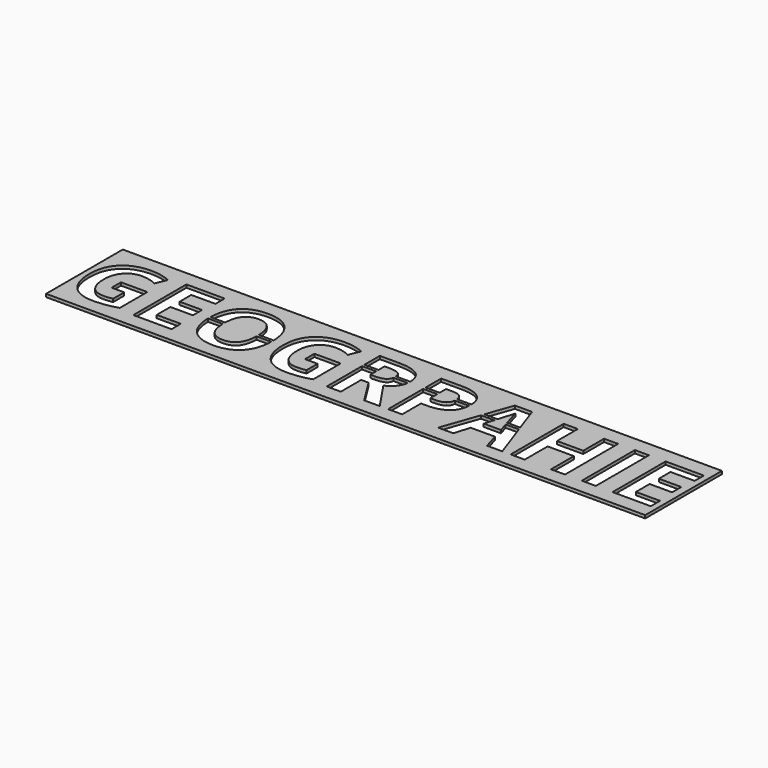
from build123d import *

# Parameters (mm, degrees)
F0_W     = 200
F0_H     = 32
F0_W_2   = 4.6989792207
F0_H_2   = 22.1564871615
F0_H_3   = 1
F1_DEPTH = 1


# Not quite as in the source:
# - a feature names something its author has since deleted; it is built from what else it names


with BuildPart() as f1:
    # F0 (on Top) → F1 (new body)
    with BuildSketch(Plane.XY):
        with Locations((100, 16)):
            Rectangle(F0_W, F0_H)
        with BuildLine():
            Line((11.1970516209, 13.3571272701), (11.1970516209, 17.2705186335))
            Line((11.1970516209, 17.2705186335), (19.9888465921, 17.2705186335))
            Line((19.9888465921, 17.2705186335), (19.9888465921, 5.7825085469))
            add(Edge.make_bspline(
                [(19.9888465921, 5.7825085469), (17.8503018694, 5.0842082293), (15.9639211503, 4.8029483791)],
                knots=[0, 0, 0, 1, 1, 1], degree=2))
            add(Edge.make_bspline(
                [(15.9639211503, 4.8029483791), (14.0775404311, 4.521688529), (12.10872148, 4.521688529)],
                knots=[0, 0, 0, 1, 1, 1], degree=2))
            add(Edge.make_bspline(
                [(12.10872148, 4.521688529), (7.0945372548, 4.521688529), (4.449239871, 7.4700676478)],
                knots=[0, 0, 0, 1, 1, 1], degree=2))
            add(Edge.make_bspline(
                [(4.449239871, 7.4700676478), (1.8039424872, 10.4184467667), (1.8039424872, 15.9369589991)],
                knots=[0, 0, 0, 1, 1, 1], degree=2))
            add(Edge.make_bspline(
                [(1.8039424872, 15.9369589991), (1.8039424872, 21.3002933831), (4.8735543001, 24.2995902335)],
                knots=[0, 0, 0, 1, 1, 1], degree=2))
            add(Edge.make_bspline(
                [(4.8735543001, 24.2995902335), (7.943166113, 27.2988870839), (13.3792401135, 27.2988870839)],
                knots=[0, 0, 0, 1, 1, 1], degree=2))
            add(Edge.make_bspline(
                [(13.3792401135, 27.2988870839), (16.7931527774, 27.2988870839), (19.9597507456, 25.9362316029)],
                knots=[0, 0, 0, 1, 1, 1], degree=2))
            Line((19.9597507456, 25.9362316029), (18.3982736464, 22.1780180879))
            add(Edge.make_bspline(
                [(18.3982736464, 22.1780180879), (15.9736197658, 23.3903450282), (13.3501442669, 23.3903450282)],
                knots=[0, 0, 0, 1, 1, 1], degree=2))
            add(Edge.make_bspline(
                [(13.3501442669, 23.3903450282), (10.3047789928, 23.3903450282), (8.471740659, 21.343937153)],
                knots=[0, 0, 0, 1, 1, 1], degree=2))
            add(Edge.make_bspline(
                [(8.471740659, 21.343937153), (6.6387023252, 19.2975292777), (6.6387023252, 15.8448221516)],
                knots=[0, 0, 0, 1, 1, 1], degree=2))
            add(Edge.make_bspline(
                [(6.6387023252, 15.8448221516), (6.6387023252, 12.2369371772), (8.1153165386, 10.3360085348)],
                knots=[0, 0, 0, 1, 1, 1], degree=2))
            add(Edge.make_bspline(
                [(8.1153165386, 10.3360085348), (9.5919307519, 8.4350798923), (12.4093785612, 8.4350798923)],
                knots=[0, 0, 0, 1, 1, 1], degree=2))
            add(Edge.make_bspline(
                [(12.4093785612, 8.4350798923), (13.8835681207, 8.4350798923), (15.3965521422, 8.7357369735)],
                knots=[0, 0, 0, 1, 1, 1], degree=2))
            Line((15.3965521422, 8.7357369735), (15.3965521422, 13.3571272701))
            Line((15.3965521422, 13.3571272701), (11.1970516209, 13.3571272701))
        make_face(mode=Mode.SUBTRACT)
        Polygon((38.0185728487, 8.706641127), (38.0185728487, 4.8271949179), (25.2600441287, 4.8271949179), (25.2600441287, 26.9836820794), (38.0185728487, 26.9836820794), (38.0185728487, 23.1333317169), (29.9590233494, 23.1333317169), (29.9590233494, 18.2694760323), (37.4609024562, 18.2694760323), (37.4609024562, 14.4191256698), (29.9590233494, 14.4191256698), (29.9590233494, 8.706641127), align=None, mode=Mode.SUBTRACT)
        with BuildLine():
            add(Edge.make_bspline(
                [(41.6555536697, 15.9660548457), (41.6555536697, 16.236144344), (41.6620706058, 16.5)],
                knots=[0, 0, 0, 0.048813765, 0.048813765, 0.048813765], degree=2))
            add(Edge.make_bspline(
                [(41.6620706058, 16.5), (41.7890597846, 21.6414978525), (44.3905632471, 24.4159736198)],
                knots=[0.048813765, 0.048813765, 0.048813765, 1, 1, 1], degree=2))
            add(Edge.make_bspline(
                [(44.3905632471, 24.4159736198), (47.1255728245, 27.3328322382), (52.2318938971, 27.3328322382)],
                knots=[0, 0, 0, 1, 1, 1], degree=2))
            add(Edge.make_bspline(
                [(52.2318938971, 27.3328322382), (57.3382149698, 27.3328322382), (60.0441287006, 24.391727081)],
                knots=[0, 0, 0, 1, 1, 1], degree=2))
            add(Edge.make_bspline(
                [(60.0441287006, 24.391727081), (62.61019587, 21.6026236075), (62.7428149058, 16.5)],
                knots=[0, 0, 0, 0.9483181744, 0.9483181744, 0.9483181744], degree=2))
            add(Edge.make_bspline(
                [(62.7428149058, 16.5), (62.7500424314, 16.2219151647), (62.7500424314, 15.9369589991)],
                knots=[0.9483181744, 0.9483181744, 0.9483181744, 1, 1, 1], degree=2))
            add(Edge.make_bspline(
                [(62.7500424314, 15.9369589991), (62.7500424314, 15.7164340599), (62.7456635168, 15.5)],
                knots=[0, 0, 0, 0.0400665642, 0.0400665642, 0.0400665642], degree=2))
            add(Edge.make_bspline(
                [(62.7456635168, 15.5), (62.6407514373, 10.3145718262), (60.0223068157, 7.4773416095)],
                knots=[0.0400665642, 0.0400665642, 0.0400665642, 1, 1, 1], degree=2))
            add(Edge.make_bspline(
                [(60.0223068157, 7.4773416095), (57.2945712, 4.521688529), (52.2027980506, 4.521688529)],
                knots=[0, 0, 0, 1, 1, 1], degree=2))
            add(Edge.make_bspline(
                [(52.2027980506, 4.521688529), (47.1110249012, 4.521688529), (44.3832892855, 7.4773416095)],
                knots=[0, 0, 0, 1, 1, 1], degree=2))
            add(Edge.make_bspline(
                [(44.3832892855, 7.4773416095), (41.7715830671, 10.3072703918), (41.6604891998, 15.5)],
                knots=[0, 0, 0, 0.9574631072, 0.9574631072, 0.9574631072], degree=2))
            add(Edge.make_bspline(
                [(41.6604891998, 15.5), (41.6555536697, 15.7306956591), (41.6555536697, 15.9660548457)],
                knots=[0.9574631072, 0.9574631072, 0.9574631072, 1, 1, 1], degree=2))
        make_face(mode=Mode.SUBTRACT)
        with BuildLine():
            Line((75.7510365395, 13.3571272701), (75.7510365395, 17.2705186335))
            Line((75.7510365395, 17.2705186335), (84.5428315108, 17.2705186335))
            Line((84.5428315108, 17.2705186335), (84.5428315108, 5.7825085469))
            add(Edge.make_bspline(
                [(84.5428315108, 5.7825085469), (82.4042867881, 5.0842082293), (80.5179060689, 4.8029483791)],
                knots=[0, 0, 0, 1, 1, 1], degree=2))
            add(Edge.make_bspline(
                [(80.5179060689, 4.8029483791), (78.6315253498, 4.521688529), (76.6627063987, 4.521688529)],
                knots=[0, 0, 0, 1, 1, 1], degree=2))
            add(Edge.make_bspline(
                [(76.6627063987, 4.521688529), (71.6485221735, 4.521688529), (69.0032247897, 7.4700676478)],
                knots=[0, 0, 0, 1, 1, 1], degree=2))
            add(Edge.make_bspline(
                [(69.0032247897, 7.4700676478), (66.3579274059, 10.4184467667), (66.3579274059, 15.9369589991)],
                knots=[0, 0, 0, 1, 1, 1], degree=2))
            add(Edge.make_bspline(
                [(66.3579274059, 15.9369589991), (66.3579274059, 21.3002933831), (69.4275392188, 24.2995902335)],
                knots=[0, 0, 0, 1, 1, 1], degree=2))
            add(Edge.make_bspline(
                [(69.4275392188, 24.2995902335), (72.4971510317, 27.2988870839), (77.9332250321, 27.2988870839)],
                knots=[0, 0, 0, 1, 1, 1], degree=2))
            add(Edge.make_bspline(
                [(77.9332250321, 27.2988870839), (81.3471376961, 27.2988870839), (84.5137356642, 25.9362316029)],
                knots=[0, 0, 0, 1, 1, 1], degree=2))
            Line((84.5137356642, 25.9362316029), (82.9522585651, 22.1780180879))
            add(Edge.make_bspline(
                [(82.9522585651, 22.1780180879), (80.5276046844, 23.3903450282), (77.9041291856, 23.3903450282)],
                knots=[0, 0, 0, 1, 1, 1], degree=2))
            add(Edge.make_bspline(
                [(77.9041291856, 23.3903450282), (74.8587639115, 23.3903450282), (73.0257255777, 21.343937153)],
                knots=[0, 0, 0, 1, 1, 1], degree=2))
            add(Edge.make_bspline(
                [(73.0257255777, 21.343937153), (71.1926872439, 19.2975292777), (71.1926872439, 15.8448221516)],
                knots=[0, 0, 0, 1, 1, 1], degree=2))
            add(Edge.make_bspline(
                [(71.1926872439, 15.8448221516), (71.1926872439, 12.2369371772), (72.6693014572, 10.3360085348)],
                knots=[0, 0, 0, 1, 1, 1], degree=2))
            add(Edge.make_bspline(
                [(72.6693014572, 10.3360085348), (74.1459156705, 8.4350798923), (76.9633634799, 8.4350798923)],
                knots=[0, 0, 0, 1, 1, 1], degree=2))
            add(Edge.make_bspline(
                [(76.9633634799, 8.4350798923), (78.4375530393, 8.4350798923), (79.9505370608, 8.7357369735)],
                knots=[0, 0, 0, 1, 1, 1], degree=2))
            Line((79.9505370608, 8.7357369735), (79.9505370608, 13.3571272701))
            Line((79.9505370608, 13.3571272701), (75.7510365395, 13.3571272701))
        make_face(mode=Mode.SUBTRACT)
        with BuildLine():
            Line((89.8140290474, 19.5501047075), (89.8140290474, 20.5501047075))
            Line((89.8140290474, 20.5501047075), (89.8140290474, 26.9836820794))
            Line((89.8140290474, 26.9836820794), (96.2684576777, 26.9836820794))
            add(Edge.make_bspline(
                [(96.2684576777, 26.9836820794), (100.7880125112, 26.9836820794), (102.9532284266, 25.3397667483)],
                knots=[0, 0, 0, 1, 1, 1], degree=2))
            add(Edge.make_bspline(
                [(102.9532284266, 25.3397667483), (105.0516471946, 23.7465663847), (105.1163836428, 20.5501047075)],
                knots=[0, 0, 0, 0.9691498908, 0.9691498908, 0.9691498908], degree=2))
            add(Edge.make_bspline(
                [(105.1163836428, 20.5501047075), (105.1184443421, 20.4483545109), (105.1184443421, 20.3449797541)],
                knots=[0.9691498908, 0.9691498908, 0.9691498908, 1, 1, 1], degree=2))
            add(Edge.make_bspline(
                [(105.1184443421, 20.3449797541), (105.1184443421, 19.9381923705), (105.0719051499, 19.5501047075)],
                knots=[0, 0, 0, 0.2081530033, 0.2081530033, 0.2081530033], degree=2))
            add(Edge.make_bspline(
                [(105.0719051499, 19.5501047075), (104.8948626908, 18.0737577624), (104.0443226729, 16.8680260893)],
                knots=[0.2081530033, 0.2081530033, 0.2081530033, 1, 1, 1], degree=2))
            add(Edge.make_bspline(
                [(104.0443226729, 16.8680260893), (102.9702010038, 15.3453434522), (100.996532745, 14.4821666707)],
                knots=[0, 0, 0, 1, 1, 1], degree=2))
            add(Edge.make_bspline(
                [(100.996532745, 14.4821666707), (106.0010183546, 7.0093834105), (107.5140023762, 4.8271949179)],
                knots=[0, 0, 0, 1, 1, 1], degree=2))
            Line((107.5140023762, 4.8271949179), (102.3009965327, 4.8271949179))
            Line((102.3009965327, 4.8271949179), (97.0104017651, 13.3280314235))
            Line((97.0104017651, 13.3280314235), (94.5130082681, 13.3280314235))
            Line((94.5130082681, 13.3280314235), (94.5130082681, 4.8271949179))
            Line((94.5130082681, 4.8271949179), (89.8140290474, 4.8271949179))
            Line((89.8140290474, 4.8271949179), (89.8140290474, 19.5501047075))
        make_face(mode=Mode.SUBTRACT)
        with BuildLine():
            Line((110.3023543389, 19.4673790485), (110.3023543389, 20.4673790485))
            Line((110.3023543389, 20.4673790485), (110.3023543389, 26.9836820794))
            Line((110.3023543389, 26.9836820794), (117.3774943627, 26.9836820794))
            add(Edge.make_bspline(
                [(117.3774943627, 26.9836820794), (121.4121184201, 26.9836820794), (123.5094440269, 25.2476299008)],
                knots=[0, 0, 0, 1, 1, 1], degree=2))
            add(Edge.make_bspline(
                [(123.5094440269, 25.2476299008), (125.484854695, 23.6124922842), (125.5996828693, 20.4673790485)],
                knots=[0, 0, 0, 0.9418712391, 0.9418712391, 0.9418712391], degree=2))
            add(Edge.make_bspline(
                [(125.5996828693, 20.4673790485), (125.6067696336, 20.2732744537), (125.6067696336, 20.0734185195)],
                knots=[0.9418712391, 0.9418712391, 0.9418712391, 1, 1, 1], degree=2))
            add(Edge.make_bspline(
                [(125.6067696336, 20.0734185195), (125.6067696336, 19.7641047233), (125.5900699964, 19.4673790485)],
                knots=[0, 0, 0, 0.0864297351, 0.0864297351, 0.0864297351], degree=2))
            add(Edge.make_bspline(
                [(125.5900699964, 19.4673790485), (125.4135532921, 16.3309613193), (123.3712387557, 14.6009747109)],
                knots=[0.0864297351, 0.0864297351, 0.0864297351, 1, 1, 1], degree=2))
            add(Edge.make_bspline(
                [(123.3712387557, 14.6009747109), (121.1357078777, 12.7073200301), (117.0137962806, 12.7073200301)],
                knots=[0, 0, 0, 1, 1, 1], degree=2))
            Line((117.0137962806, 12.7073200301), (115.0013335596, 12.7073200301))
            Line((115.0013335596, 12.7073200301), (115.0013335596, 4.8271949179))
            Line((115.0013335596, 4.8271949179), (110.3023543389, 4.8271949179))
            Line((110.3023543389, 4.8271949179), (110.3023543389, 19.4673790485))
        make_face(mode=Mode.SUBTRACT)
        Polygon((131.3632866146, 17.2284944803), (131.7148559258, 18.2284944803), (134.8253036879, 27.0758189268), (140.5668840773, 27.0758189268), (143.6889020108, 18.2284944803), (144.0417790814, 17.2284944803), (148.4179133429, 4.8271949179), (143.3552360401, 4.8271949179), (141.7501151711, 10.1032417622), (133.6711684407, 10.1032417622), (132.0660475717, 4.8271949179), (127.0033702689, 4.8271949179), align=None, mode=Mode.SUBTRACT)
        Polygon((169.362073564, 26.9836820794), (169.362073564, 4.8271949179), (164.6776422666, 4.8271949179), (164.6776422666, 14.3900298232), (155.9052445263, 14.3900298232), (155.9052445263, 4.8271949179), (151.2062653056, 4.8271949179), (151.2062653056, 26.9836820794), (155.9052445263, 26.9836820794), (155.9052445263, 18.2985718789), (164.6776422666, 18.2985718789), (164.6776422666, 26.9836820794), align=None, mode=Mode.SUBTRACT)
        with Locations((177.3028150232, 15.9054384987)):
            Rectangle(F0_W_2, F0_H_2, mode=Mode.SUBTRACT)
        Polygon((197.9875372791, 8.706641127), (197.9875372791, 4.8271949179), (185.229008559, 4.8271949179), (185.229008559, 26.9836820794), (197.9875372791, 26.9836820794), (197.9875372791, 23.1333317169), (189.9279877797, 23.1333317169), (189.9279877797, 18.2694760323), (197.4298668865, 18.2694760323), (197.4298668865, 14.4191256698), (189.9279877797, 14.4191256698), (189.9279877797, 8.706641127), align=None, mode=Mode.SUBTRACT)
        with BuildLine():
            Line((57.8181957487, 15.5), (46.5874707337, 15.5))
            add(Edge.make_bspline(
                [(46.5874707337, 15.5), (46.6665474848, 12.1102114993), (47.9911742599, 10.3432824964)],
                knots=[0.0596973824, 0.0596973824, 0.0596973824, 1, 1, 1], degree=2))
            add(Edge.make_bspline(
                [(47.9911742599, 10.3432824964), (49.3998981645, 8.4641757389), (52.2027980506, 8.4641757389)],
                knots=[0, 0, 0, 1, 1, 1], degree=2))
            add(Edge.make_bspline(
                [(52.2027980506, 8.4641757389), (57.656350345, 8.4641757389), (57.8181957487, 15.5)],
                knots=[0, 0, 0, 0.9703229391, 0.9703229391, 0.9703229391], degree=2))
        make_face()
        with BuildLine():
            add(Edge.make_bspline(
                [(48.0057221832, 21.5330601557), (46.6925516643, 19.7926058735), (46.5909675604, 16.5)],
                knots=[0, 0, 0, 0.9226421075, 0.9226421075, 0.9226421075], degree=2))
            Line((46.5909675604, 16.5), (57.8149184145, 16.5))
            add(Edge.make_bspline(
                [(57.8149184145, 16.5), (57.6086671178, 23.4194408748), (52.2318938971, 23.4194408748)],
                knots=[0.0383596794, 0.0383596794, 0.0383596794, 1, 1, 1], degree=2))
            add(Edge.make_bspline(
                [(52.2318938971, 23.4194408748), (49.4289940111, 23.4194408748), (48.0057221832, 21.5330601557)],
                knots=[0, 0, 0, 1, 1, 1], degree=2))
        make_face()
        with BuildLine():
            Line((139.6358245633, 17.2284944803), (135.8330191332, 17.2284944803))
            add(Edge.make_bspline(
                [(135.8330191332, 17.2284944803), (135.3919484767, 15.7826706927), (134.8543995345, 14.0408796644)],
                knots=[0.772380585, 0.772380585, 0.772380585, 1, 1, 1], degree=2))
            Line((134.8543995345, 14.0408796644), (140.6250757704, 14.0408796644))
            add(Edge.make_bspline(
                [(140.6250757704, 14.0408796644), (140.0699793007, 15.8283144841), (139.6358245633, 17.2284944803)],
                knots=[0, 0, 0, 0.2493882756, 0.2493882756, 0.2493882756], degree=2))
        make_face()
        with BuildLine():
            Line((120.8436359326, 19.4673790485), (115.0013335596, 19.4673790485))
            Line((115.0013335596, 19.4673790485), (115.0013335596, 16.5576703926))
            Line((115.0013335596, 16.5576703926), (116.5482627355, 16.5576703926))
            add(Edge.make_bspline(
                [(116.5482627355, 16.5576703926), (118.711053997, 16.5576703926), (119.7876003201, 17.4135732124)],
                knots=[0, 0, 0, 1, 1, 1], degree=2))
            add(Edge.make_bspline(
                [(119.7876003201, 17.4135732124), (120.7155507821, 18.1513356293), (120.8436359326, 19.4673790485)],
                knots=[0, 0, 0, 0.8619698402, 0.8619698402, 0.8619698402], degree=2))
        make_face()
        with BuildLine():
            Line((115.0013335596, 23.1333317169), (115.0013335596, 20.4673790485))
            Line((115.0013335596, 20.4673790485), (120.8353082496, 20.4673790485))
            add(Edge.make_bspline(
                [(120.8353082496, 20.4673790485), (120.702866137, 21.6982103624), (119.9621753995, 22.3453192057)],
                knots=[0.1788089224, 0.1788089224, 0.1788089224, 1, 1, 1], degree=2))
            add(Edge.make_bspline(
                [(119.9621753995, 22.3453192057), (119.0602041559, 23.1333317169), (117.1350289746, 23.1333317169)],
                knots=[0, 0, 0, 1, 1, 1], degree=2))
            Line((117.1350289746, 23.1333317169), (115.0013335596, 23.1333317169))
        make_face()
        with BuildLine():
            Line((94.5130082681, 23.1333317169), (94.5130082681, 20.5501047075))
            Line((94.5130082681, 20.5501047075), (100.3634520099, 20.5501047075))
            add(Edge.make_bspline(
                [(100.3634520099, 20.5501047075), (100.2600364504, 21.8710044043), (99.2920010668, 22.4665518997)],
                knots=[0.1068303507, 0.1068303507, 0.1068303507, 1, 1, 1], degree=2))
            add(Edge.make_bspline(
                [(99.2920010668, 22.4665518997), (98.2081807822, 23.1333317169), (95.9387047499, 23.1333317169)],
                knots=[0, 0, 0, 1, 1, 1], degree=2))
            Line((95.9387047499, 23.1333317169), (94.5130082681, 23.1333317169))
        make_face()
        with BuildLine():
            Line((100.3220361566, 19.5501047075), (94.5130082681, 19.5501047075))
            Line((94.5130082681, 19.5501047075), (94.5130082681, 17.1492859394))
            Line((94.5130082681, 17.1492859394), (96.0259922896, 17.1492859394))
            add(Edge.make_bspline(
                [(96.0259922896, 17.1492859394), (98.2566738598, 17.1492859394), (99.3162476057, 17.8912300269)],
                knots=[0, 0, 0, 1, 1, 1], degree=2))
            add(Edge.make_bspline(
                [(99.3162476057, 17.8912300269), (100.137096865, 18.4660123458), (100.3220361566, 19.5501047075)],
                knots=[0, 0, 0, 0.7746976202, 0.7746976202, 0.7746976202], degree=2))
        make_face()
        with BuildLine():
            Line((57.8149184145, 16.5), (46.5909675604, 16.5))
            add(Edge.make_bspline(
                [(46.5909675604, 16.5), (46.5824503552, 16.223935154), (46.5824503552, 15.9369589991)],
                knots=[0.9226421075, 0.9226421075, 0.9226421075, 1, 1, 1], degree=2))
            add(Edge.make_bspline(
                [(46.5824503552, 15.9369589991), (46.5824503552, 15.7152089087), (46.5874707337, 15.5)],
                knots=[0, 0, 0, 0.0596973824, 0.0596973824, 0.0596973824], degree=2))
            Line((46.5874707337, 15.5), (57.8181957487, 15.5))
            add(Edge.make_bspline(
                [(57.8181957487, 15.5), (57.8231457459, 15.715188755), (57.8231457459, 15.9369589991)],
                knots=[0.9703229391, 0.9703229391, 0.9703229391, 1, 1, 1], degree=2))
            add(Edge.make_bspline(
                [(57.8231457459, 15.9369589991), (57.8231457459, 16.2239846046), (57.8149184145, 16.5)],
                knots=[0, 0, 0, 0.0383596794, 0.0383596794, 0.0383596794], degree=2))
        make_face()
        with BuildLine():
            add(Edge.make_bspline(
                [(137.7154911136, 23.6328104163), (137.3705203782, 22.2931182399), (136.1372867158, 18.2284944803)],
                knots=[0, 0, 0, 0.6906615554, 0.6906615554, 0.6906615554], degree=2))
            Line((136.1372867158, 18.2284944803), (139.3258767157, 18.2284944803))
            add(Edge.make_bspline(
                [(139.3258767157, 18.2284944803), (138.3026761722, 21.5311576243), (138.1179836578, 22.1489222414)],
                knots=[0.3433385026, 0.3433385026, 0.3433385026, 1, 1, 1], degree=2))
            add(Edge.make_bspline(
                [(138.1179836578, 22.1489222414), (137.8367238077, 23.089687947), (137.7154911136, 23.6328104163)],
                knots=[0, 0, 0, 1, 1, 1], degree=2))
        make_face()
        with BuildLine():
            Line((120.8353082496, 20.4673790485), (115.0013335596, 20.4673790485))
            Line((115.0013335596, 20.4673790485), (115.0013335596, 19.4673790485))
            Line((115.0013335596, 19.4673790485), (120.8436359326, 19.4673790485))
            add(Edge.make_bspline(
                [(120.8436359326, 19.4673790485), (120.8641466431, 19.6781215535), (120.8641466431, 19.9036927479)],
                knots=[0.8619698402, 0.8619698402, 0.8619698402, 1, 1, 1], degree=2))
            add(Edge.make_bspline(
                [(120.8641466431, 19.9036927479), (120.8641466431, 20.1993736757), (120.8353082496, 20.4673790485)],
                knots=[0, 0, 0, 0.1788089224, 0.1788089224, 0.1788089224], degree=2))
        make_face()
        with BuildLine():
            Line((100.3634520099, 20.5501047075), (94.5130082681, 20.5501047075))
            Line((94.5130082681, 20.5501047075), (94.5130082681, 19.5501047075))
            Line((94.5130082681, 19.5501047075), (100.3220361566, 19.5501047075))
            add(Edge.make_bspline(
                [(100.3220361566, 19.5501047075), (100.3758213515, 19.8653871902), (100.3758213515, 20.2237470601)],
                knots=[0.7746976202, 0.7746976202, 0.7746976202, 1, 1, 1], degree=2))
            add(Edge.make_bspline(
                [(100.3758213515, 20.2237470601), (100.3758213515, 20.392114366), (100.3634520099, 20.5501047075)],
                knots=[0, 0, 0, 0.1068303507, 0.1068303507, 0.1068303507], degree=2))
        make_face()
        with BuildLine():
            Line((46.5909675604, 16.5), (41.6620706058, 16.5))
            add(Edge.make_bspline(
                [(41.6555536697, 15.9660548457), (41.6555536697, 16.236144344), (41.6620706058, 16.5)],
                knots=[0, 0, 0, 0.048813765, 0.048813765, 0.048813765], degree=2))
            add(Edge.make_bspline(
                [(41.6604891998, 15.5), (41.6555536697, 15.7306956591), (41.6555536697, 15.9660548457)],
                knots=[0.9574631072, 0.9574631072, 0.9574631072, 1, 1, 1], degree=2))
            Line((41.6604891998, 15.5), (46.5874707337, 15.5))
            add(Edge.make_bspline(
                [(46.5824503552, 15.9369589991), (46.5824503552, 15.7152089087), (46.5874707337, 15.5)],
                knots=[0, 0, 0, 0.0596973824, 0.0596973824, 0.0596973824], degree=2))
            add(Edge.make_bspline(
                [(46.5909675604, 16.5), (46.5824503552, 16.223935154), (46.5824503552, 15.9369589991)],
                knots=[0.9226421075, 0.9226421075, 0.9226421075, 1, 1, 1], degree=2))
        make_face()
        with BuildLine():
            Line((62.7428149058, 16.5), (57.8149184145, 16.5))
            add(Edge.make_bspline(
                [(57.8231457459, 15.9369589991), (57.8231457459, 16.2239846046), (57.8149184145, 16.5)],
                knots=[0, 0, 0, 0.0383596794, 0.0383596794, 0.0383596794], degree=2))
            add(Edge.make_bspline(
                [(57.8181957487, 15.5), (57.8231457459, 15.715188755), (57.8231457459, 15.9369589991)],
                knots=[0.9703229391, 0.9703229391, 0.9703229391, 1, 1, 1], degree=2))
            Line((57.8181957487, 15.5), (62.7456635168, 15.5))
            add(Edge.make_bspline(
                [(62.7500424314, 15.9369589991), (62.7500424314, 15.7164340599), (62.7456635168, 15.5)],
                knots=[0, 0, 0, 0.0400665642, 0.0400665642, 0.0400665642], degree=2))
            add(Edge.make_bspline(
                [(62.7428149058, 16.5), (62.7500424314, 16.2219151647), (62.7500424314, 15.9369589991)],
                knots=[0.9483181744, 0.9483181744, 0.9483181744, 1, 1, 1], degree=2))
        make_face()
        with BuildLine():
            Line((125.5996828693, 20.4673790485), (120.8353082496, 20.4673790485))
            add(Edge.make_bspline(
                [(120.8641466431, 19.9036927479), (120.8641466431, 20.1993736757), (120.8353082496, 20.4673790485)],
                knots=[0, 0, 0, 0.1788089224, 0.1788089224, 0.1788089224], degree=2))
            add(Edge.make_bspline(
                [(120.8436359326, 19.4673790485), (120.8641466431, 19.6781215535), (120.8641466431, 19.9036927479)],
                knots=[0.8619698402, 0.8619698402, 0.8619698402, 1, 1, 1], degree=2))
            Line((120.8436359326, 19.4673790485), (125.5900699964, 19.4673790485))
            add(Edge.make_bspline(
                [(125.6067696336, 20.0734185195), (125.6067696336, 19.7641047233), (125.5900699964, 19.4673790485)],
                knots=[0, 0, 0, 0.0864297351, 0.0864297351, 0.0864297351], degree=2))
            add(Edge.make_bspline(
                [(125.5996828693, 20.4673790485), (125.6067696336, 20.2732744537), (125.6067696336, 20.0734185195)],
                knots=[0.9418712391, 0.9418712391, 0.9418712391, 1, 1, 1], degree=2))
        make_face()
        with BuildLine():
            Line((105.1163836428, 20.5501047075), (100.3634520099, 20.5501047075))
            add(Edge.make_bspline(
                [(100.3758213515, 20.2237470601), (100.3758213515, 20.392114366), (100.3634520099, 20.5501047075)],
                knots=[0, 0, 0, 0.1068303507, 0.1068303507, 0.1068303507], degree=2))
            add(Edge.make_bspline(
                [(100.3220361566, 19.5501047075), (100.3758213515, 19.8653871902), (100.3758213515, 20.2237470601)],
                knots=[0.7746976202, 0.7746976202, 0.7746976202, 1, 1, 1], degree=2))
            Line((100.3220361566, 19.5501047075), (105.0719051499, 19.5501047075))
            add(Edge.make_bspline(
                [(105.1184443421, 20.3449797541), (105.1184443421, 19.9381923705), (105.0719051499, 19.5501047075)],
                knots=[0, 0, 0, 0.2081530033, 0.2081530033, 0.2081530033], degree=2))
            add(Edge.make_bspline(
                [(105.1163836428, 20.5501047075), (105.1184443421, 20.4483545109), (105.1184443421, 20.3449797541)],
                knots=[0.9691498908, 0.9691498908, 0.9691498908, 1, 1, 1], degree=2))
        make_face()
        with Locations((92.1635186577, 20.0501047075)):
            Rectangle(F0_W_2, F0_H_3)
        with Locations((112.6518439493, 19.9673790485)):
            Rectangle(F0_W_2, F0_H_3)
        with BuildLine():
            Line((136.1372867158, 18.2284944803), (131.7148559258, 18.2284944803))
            Line((131.7148559258, 18.2284944803), (131.3632866146, 17.2284944803))
            Line((131.3632866146, 17.2284944803), (135.8330191332, 17.2284944803))
            add(Edge.make_bspline(
                [(136.1372867158, 18.2284944803), (135.9913705904, 17.7475684656), (135.8330191332, 17.2284944803)],
                knots=[0.6906615554, 0.6906615554, 0.6906615554, 0.772380585, 0.772380585, 0.772380585], degree=2))
        make_face()
        with BuildLine():
            Line((143.6889020108, 18.2284944803), (139.3258767157, 18.2284944803))
            add(Edge.make_bspline(
                [(139.6358245633, 17.2284944803), (139.4722686141, 17.7559740825), (139.3258767157, 18.2284944803)],
                knots=[0.2493882756, 0.2493882756, 0.2493882756, 0.3433385026, 0.3433385026, 0.3433385026], degree=2))
            Line((139.6358245633, 17.2284944803), (144.0417790814, 17.2284944803))
            Line((144.0417790814, 17.2284944803), (143.6889020108, 18.2284944803))
        make_face()
        with BuildLine():
            Line((139.3258767157, 18.2284944803), (136.1372867158, 18.2284944803))
            add(Edge.make_bspline(
                [(136.1372867158, 18.2284944803), (135.9913705904, 17.7475684656), (135.8330191332, 17.2284944803)],
                knots=[0.6906615554, 0.6906615554, 0.6906615554, 0.772380585, 0.772380585, 0.772380585], degree=2))
            Line((135.8330191332, 17.2284944803), (139.6358245633, 17.2284944803))
            add(Edge.make_bspline(
                [(139.6358245633, 17.2284944803), (139.4722686141, 17.7559740825), (139.3258767157, 18.2284944803)],
                knots=[0.2493882756, 0.2493882756, 0.2493882756, 0.3433385026, 0.3433385026, 0.3433385026], degree=2))
        make_face()
    extrude(amount=F1_DEPTH)


solid = f1.part
